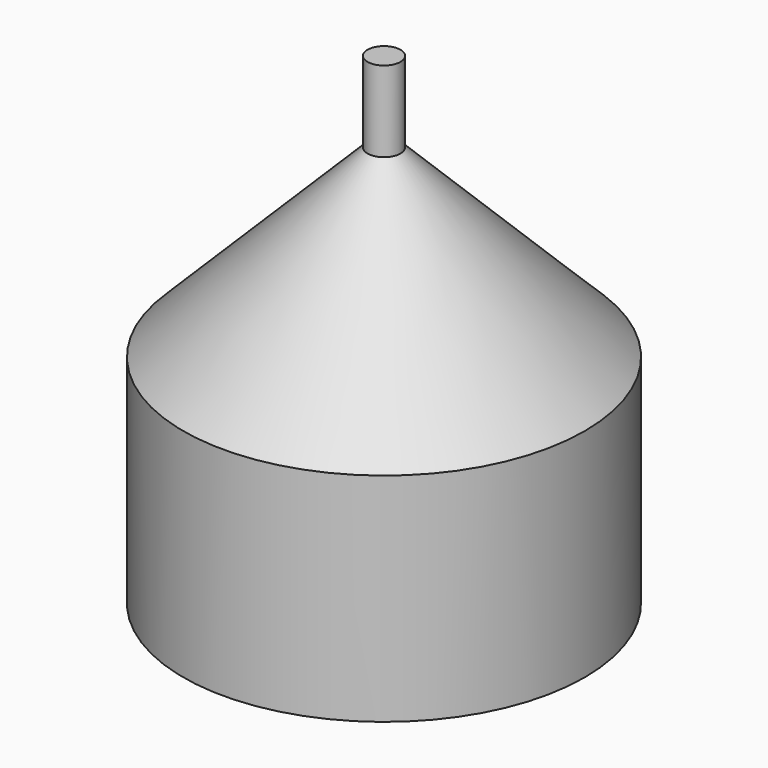
from build123d import *

# Parameters (mm, degrees)
F0_R        = 50
F1_DEPTH    = 100
F2_R        = 4.1
F3_DEPTH    = 20
F4_S5_R     = 4.1
F4_T6_DEPTH = 76


# Not quite as in the source:
# - a fillet or chamfer that OpenCascade refuses, or shapes differently, is made with other operations: its cross-section is extruded or revolved along the edge and cut away or added


with BuildPart() as f1:
    # F0 (on Top) → F1 (new body)
    with BuildSketch(Plane.XY):
        Circle(F0_R)
    extrude(amount=F1_DEPTH)

    # F2 (on face) → F3 (join)
    with BuildSketch(Plane.XY.offset(100)):
        Circle(F2_R)
    extrude(amount=F3_DEPTH)

    # F4: chamfer of 46 on 1 edges, made by hand


with BuildPart() as f4_tool2:
    # F4_s3 → F4_t4 (revolve)
    with BuildSketch(Plane.XZ):
        Polygon((50, 54), (4, 100), (50, 100), align=None)
    revolve(axis=Axis((0, 0, 100), (0, 0, 1)))

    # F4_s5 → F4_t6 (cut, symmetric)
    with BuildSketch(Plane.XY.offset(77)):
        Circle(F4_S5_R)
    extrude(amount=F4_T6_DEPTH, both=True, mode=Mode.SUBTRACT)


with BuildPart() as f1_1:
    add(f1.part)

    # F4_t1: cut F4_tool2
    add(f4_tool2.part, mode=Mode.SUBTRACT)


solid = f1_1.part
